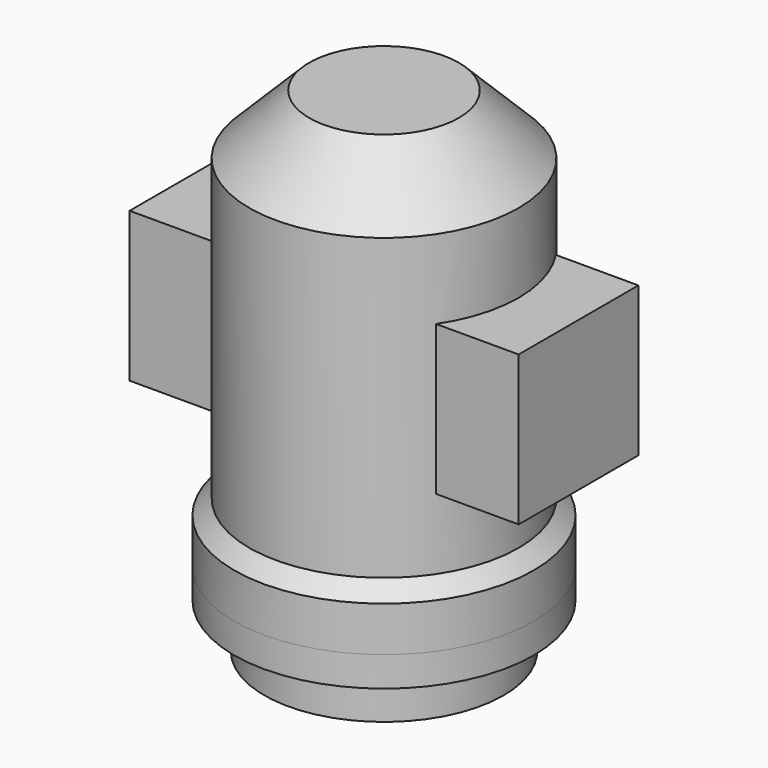
from build123d import *

# Parameters (mm, degrees)
F0_R        = 10.16
F1_DEPTH    = 3.81
F2_R        = 12.7
F3_DEPTH    = 2.54
F4_R        = 11.43
F5_DEPTH    = 38.1
F6_S5_R     = 12.7
F6_T6_DEPTH = 25
F7_W        = 12.7
F7_H        = 12.7
F8_DEPTH    = 16.51
F9_W        = 12.7
F9_H        = 12.7
F10_DEPTH   = 16.51


# Not quite as in the source:
# - a fillet or chamfer that OpenCascade refuses, or shapes differently, is made with other operations: its cross-section is extruded or revolved along the edge and cut away or added


with BuildPart() as f1:
    # F0 (on Top) → F1 (new body)
    with BuildSketch(Plane.XY):
        Circle(F0_R)
    extrude(amount=-F1_DEPTH)

    # F2 (on Top) → F3 (join)
    with BuildSketch(Plane.XY):
        Circle(F2_R)
    extrude(amount=F3_DEPTH)

    # F4 (on Top) → F5 (join)
    with BuildSketch(Plane.XY):
        Circle(F4_R)
    extrude(amount=F5_DEPTH)

    # F6: chamfer of 5.08 on 3 edges, made by hand


with BuildPart() as f6_tool2:
    # F6_s3 → F6_t4 (revolve)
    with BuildSketch(Plane.XZ):
        Polygon((16.51, 2.54), (11.43, 7.62), (11.43, 2.54), align=None)
    revolve(axis=Axis((0, 0, 2.54), (0, 0, -1)))

    # F6_s5 → F6_t6 (intersect, symmetric)
    with BuildSketch(Plane.XY.offset(5.1)):
        Circle(F6_S5_R)
    extrude(amount=F6_T6_DEPTH, both=True, mode=Mode.INTERSECT)


with BuildPart() as f1_1:
    add(f1.part)

    # F6_t1: union F6_tool2
    add(f6_tool2.part)

    # F6_s7 → F6_t8 (revolve, cut)
    with BuildSketch(Plane.XZ):
        Polygon((11.43, 33.02), (6.35, 38.1), (11.43, 38.1), align=None)
    revolve(axis=Axis((0, 0, 38.1), (0, 0, 1)), mode=Mode.SUBTRACT)

    # F7 (on Right) → F8 (join)
    with BuildSketch(Plane.YZ):
        with Locations((0, 19.9612583965)):
            Rectangle(F7_W, F7_H)
    extrude(amount=F8_DEPTH)

    # F9 (on Right) → F10 (join)
    with BuildSketch(Plane.YZ):
        with Locations((0, 19.9612583965)):
            Rectangle(F9_W, F9_H)
    extrude(amount=-F10_DEPTH)


solid = f1_1.part
